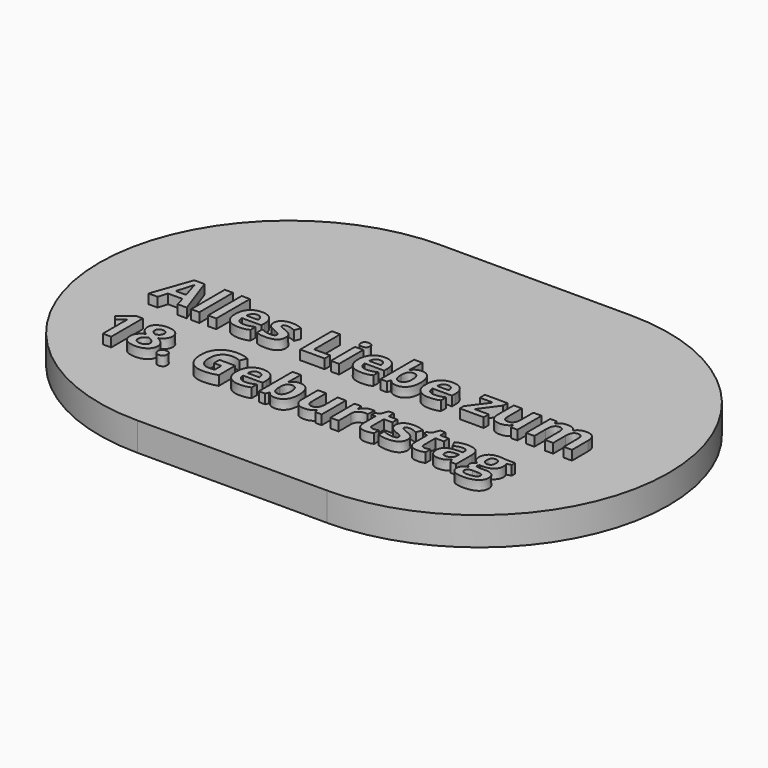
from build123d import *

# Parameters (mm, degrees)
F0_W         = 20
F0_H         = 40
F1_DEPTH     = 3
F2_TEXT_SIZE = 5.8370490474
F3_DEPTH     = 1


# Not quite as in the source:
# - Text() gives the source's letters only with a copy of the font that has no kerning and outlines rounded to 1/6400 em; it was checked with that copy


with BuildPart() as f1:
    # F0 (on Top) → F1 (new body)
    with BuildSketch(Plane.XY):
        with BuildLine():
            ThreePointArc((-10, 20), (-30, 0), (-10, -20))
            Line((-10, -20), (-10, 20))
        make_face()
        Rectangle(F0_W, F0_H)
        with BuildLine():
            Line((10, 20), (10, -20))
            ThreePointArc((10, -20), (30, 0), (10, 20))
        make_face()
    extrude(amount=F1_DEPTH)

    # F2 (on face) → F3 (join)
    with BuildSketch(Plane.XY.offset(3)):
        with Locations((-22.2091811444, -3.2516594392)):
            Text('Alles Liebe zum', F2_TEXT_SIZE, font='Open Sans', font_style=FontStyle.BOLD, text_align=(TextAlign.LEFT, TextAlign.BOTTOM))
        with Locations((-22.2091811444, -11.1900461437)):
            Text('18. Geburtstag', F2_TEXT_SIZE, font='Open Sans', font_style=FontStyle.BOLD, text_align=(TextAlign.LEFT, TextAlign.BOTTOM))
    extrude(amount=F3_DEPTH)


solid = f1.part
